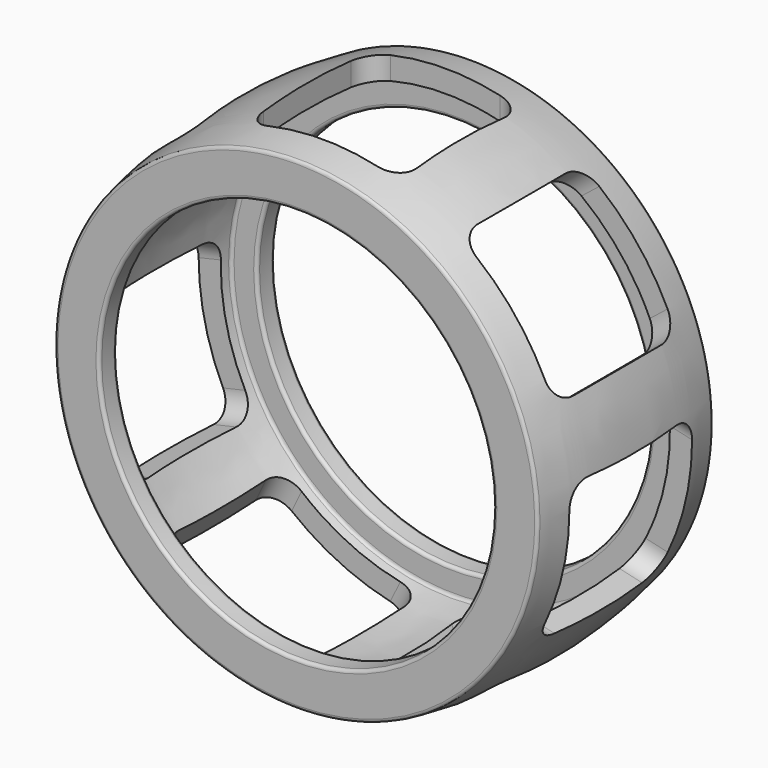
from build123d import *

# Parameters (mm, degrees)
F2_T            = -1
F3_R            = 0.15
F5_DEPTH        = 11.5061026722
F5_COPIES_COUNT = 7


# Not quite as in the source:
# - a pattern or mirror of a feature is missing from the dataset's text; its kind, count and spacing are read off the source's solid


with BuildPart() as f1:
    # F0 (on Top) → F1 (revolve)
    with BuildSketch(Plane.XY):
        with BuildLine():
            Line((-9, -5), (-9, 5))
            Line((-9, 5), (-11, 5))
            ThreePointArc((-11, 5), (-11.5051025722, 0), (-11, -5))
            Line((-11, -5), (-9, -5))
        make_face()
    revolve(axis=Axis((0, -4.8633189872, 0), (0, -1, 0)))

    # F2
    f2_openings = [f1.faces().sort_by_distance(p)[0] for p in [
        (9, 0, 0),
    ]]
    offset(amount=F2_T, openings=f2_openings, kind=Kind.INTERSECTION)

    # F3
    f3_edges = [f1.edges().sort_by_distance(p)[0] for p in [
        (9, -5, 0),
        (10.169422, 4, 0),
        (9, 4, 0),
        (9, 5, 0),
        (11, 5, 0),
        (9, -4, 0),
        (11, -5, 0),
        (10.169422, -4, 0),
        (-11.505103, 0, 0),
        (-9, 4.5, 0),
        (-9, -4.5, 0),
    ]]
    fillet(f3_edges, radius=F3_R)

    # F4 (on Top) → F5 (cut, through all)
    with BuildSketch(Plane.XY):
        with BuildLine():
            Line((-2.5, -3.5), (2.5, -3.5))
            ThreePointArc((2.5, -3.5), (3.2071067812, -3.2071067812), (3.5, -2.5))
            Line((3.5, -2.5), (3.5, 2.5))
            ThreePointArc((3.5, 2.5), (3.2071067812, 3.2071067812), (2.5, 3.5))
            Line((2.5, 3.5), (-2.5, 3.5))
            ThreePointArc((-2.5, 3.5), (-3.2071067812, 3.2071067812), (-3.5, 2.5))
            Line((-3.5, 2.5), (-3.5, -2.5))
            ThreePointArc((-3.5, -2.5), (-3.2071067812, -3.2071067812), (-2.5, -3.5))
        make_face()
    f5 = extrude(amount=F5_DEPTH, mode=Mode.SUBTRACT)

    # F5_copies: F5 ×7 about axis
    f5_copies_axis = Axis((0, 0, 0), (0, 1, 0))
    for i in range(1, F5_COPIES_COUNT):
        add(f5.rotate(f5_copies_axis, i * 360 / F5_COPIES_COUNT), mode=Mode.SUBTRACT)


solid = f1.part
